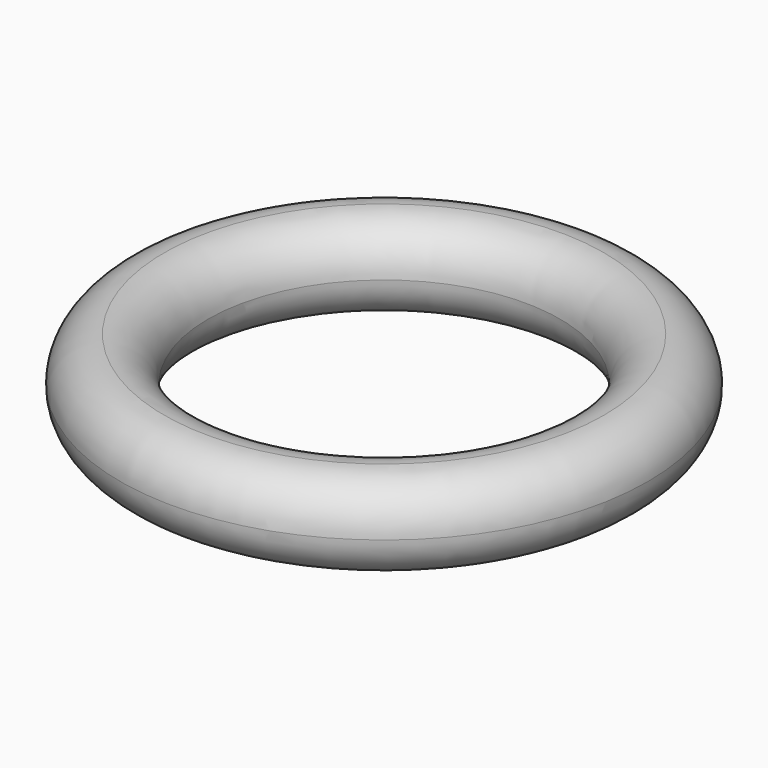
from build123d import *

# Parameters (mm, degrees)
F0_R     = 4.7625
F0_R_2   = 3.175
F1_DEPTH = 1.5875
F2_R     = 0.79374


# Not quite as in the source:
# - a fillet or chamfer is up to 0.001 mm smaller than in the source, because OpenCascade refuses the exact size


with BuildPart() as f1:
    # F0 (on Top) → F1 (new body)
    with BuildSketch(Plane.XY):
        Circle(F0_R)
        Circle(F0_R_2, mode=Mode.SUBTRACT)
    extrude(amount=F1_DEPTH)

    # F2 (radius 0.79375 in the source; OpenCascade refuses exactly that, so slightly less here)
    f2_edges = [f1.edges().sort_by_distance(p)[0] for p in [
        (-3.175, 0, 1.5875),
        (-3.175, 0, 0),
        (-4.7625, 0, 1.5875),
        (-4.7625, 0, 0),
    ]]
    fillet(f2_edges, radius=F2_R)


solid = f1.part
